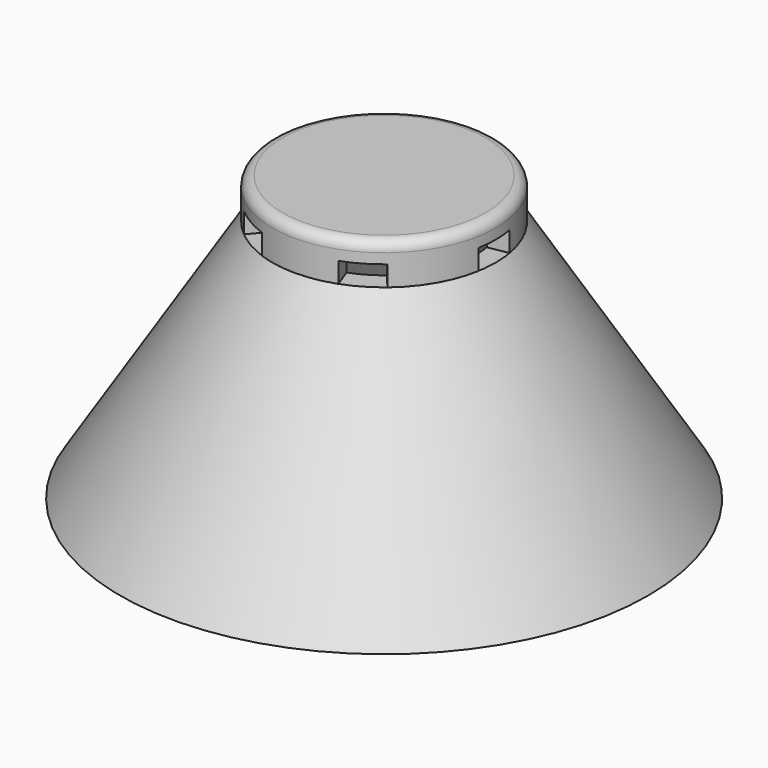
from build123d import *

# Parameters (mm, degrees)
F3_DEPTH        = 2
F5_R            = 11
F6_DEPTH        = 2
F4_W            = 2
F4_H            = 2
F7_ANGLE_BACK   = 10
F7_ANGLE        = 20
F7_COPIES_COUNT = 6
F8_R            = 1


# Not quite as in the source:
# - a pattern or mirror of a feature is missing from the dataset's text; its kind, count and spacing are read off the source's solid


with BuildPart() as f1:
    # F0 (on Front) → F1 (revolve)
    with BuildSketch(Plane.XZ):
        Polygon((11, 24), (9, 24), (24, 0), (26, 0), align=None)
    revolve(axis=Axis((0, 0, 12), (0, 0, 1)))


with BuildPart() as f3:
    # F3 (new): a face of the model
    f3_faces = [f1.part.faces().sort_by_distance(p)[0] for p in [
        (-10.6888730163, 0, 24),
    ]]
    extrude(f3_faces, amount=F3_DEPTH)

    # F5 (on face) → F6 (join)
    with BuildSketch(Plane.XY.offset(26)):
        Circle(F5_R)
    extrude(amount=F6_DEPTH)

    # F4 (on Front) → F7 (revolve, cut)
    with BuildSketch(Plane.XZ, mode=Mode.PRIVATE) as f7_sk:
        with Locations((10, 25)):
            Rectangle(F4_W, F4_H)
    f7 = revolve(f7_sk.sketch.rotate(Axis((0, 0, 28.8), (0, 0, -1)), -F7_ANGLE_BACK), axis=Axis((0, 0, 28.8), (0, 0, -1)), revolution_arc=F7_ANGLE, mode=Mode.SUBTRACT)

    # F7_copies: F7 ×6 about axis
    f7_copies_axis = Axis((0, 0, 0), (0, 0, 1))
    for i in range(1, F7_COPIES_COUNT):
        add(f7.rotate(f7_copies_axis, i * 360 / F7_COPIES_COUNT), mode=Mode.SUBTRACT)

    # F8
    f8_edges = [f3.edges().sort_by_distance(p)[0] for p in [
        (-11, 0, 28),
    ]]
    fillet(f8_edges, radius=F8_R)


solid = Compound([f1.part, f3.part])
